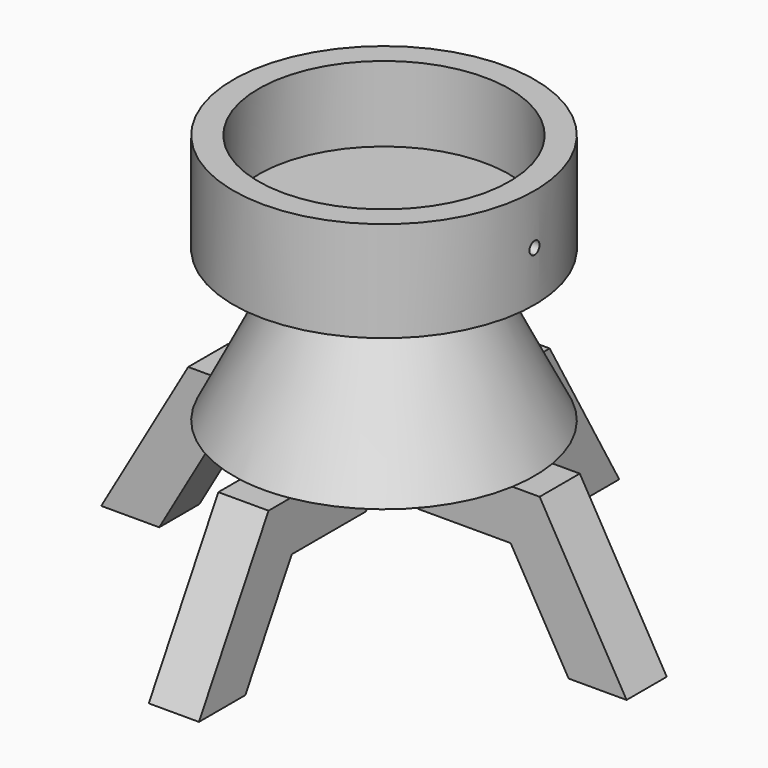
from build123d import *

# Parameters (mm, degrees)
F1_DEPTH  = 50.8
F4_DEPTH  = 50.8
F11_DEPTH = 762


with BuildPart() as f1:
    # F0 (on Front) → F1 (new body)
    with BuildSketch(Plane.XZ):
        Polygon((-320.5175746993, 101.6), (-291.1881810245, 152.4), (-443.5881810245, 152.4), (-531.576362049, 0), (-472.9175746993, 0), (-414.2587873497, 101.6), align=None)
    extrude(amount=F1_DEPTH)



with BuildPart() as f1b:
    # F0 (on Front) → F1, piece 2 (new body)
    with BuildSketch(Plane.XZ):
        Polygon((-58.6587873497, 0), (0, 0), (-87.9881810245, 152.4), (-240.3881810245, 152.4), (-211.0587873497, 101.6), (-117.3175746993, 101.6), align=None)
    extrude(amount=F1_DEPTH)


with BuildPart() as f1_1:
    add(f1.part)

    add(f1b.part)  # F4 merges F1b
    # F3 (on face) → F4 (join)
    with BuildSketch(Plane(origin=(-291.1881810245, 0, 0), x_dir=(0, -1, 0), z_dir=(-1, 0, 0))):
        Polygon((203.2, 152.4), (50.8, 152.4), (80.1293936748, 101.6), (173.8706063252, 101.6), (232.5293936748, 0), (291.1881810245, 0), align=None)
        Polygon((-29.3293936748, 101.6), (0, 152.4), (-152.4, 152.4), (-240.3881810245, 0), (-181.7293936748, 0), (-123.0706063252, 101.6), align=None)
    extrude(amount=-F4_DEPTH)

    # F7 (on face) → F9 (revolve)
    with BuildSketch(Plane(origin=(-265.7881810245, 0, 0), x_dir=(0, -1, 0), z_dir=(-1, 0, 0))):
        Polygon((25.4, 304.8), (25.4, 152.4), (177.8, 152.4), (101.6, 304.8), align=None)
    revolve(axis=Axis((-265.7881810245, -25.4, 228.6), (0, 0, 1)))

    # F7 (on face) → F10 (revolve)
    with BuildSketch(Plane(origin=(-265.7881810245, 0, 0), x_dir=(0, -1, 0), z_dir=(-1, 0, 0))):
        Polygon((25.4, 330.2), (25.4, 304.8), (101.6, 304.8), (177.8, 304.8), (177.8, 406.4), (152.4, 406.4), (152.4, 330.2), align=None)
    revolve(axis=Axis((-265.7881810245, -25.4, 330.2), (0, 0, 1)))

    # F7 (on face) → F11 (cut)
    with BuildSketch(Plane(origin=(-265.7881810245, 0, 0), x_dir=(0, -1, 0), z_dir=(-1, 0, 0))):
        with BuildLine():
            ThreePointArc((31.75, 355.6), (20.9098719395, 360.0901280605), (25.4, 349.25))
            ThreePointArc((25.4, 349.25), (29.8901280605, 351.1098719395), (31.75, 355.6))
        make_face()
    extrude(amount=-F11_DEPTH, mode=Mode.SUBTRACT)


solid = f1_1.part
